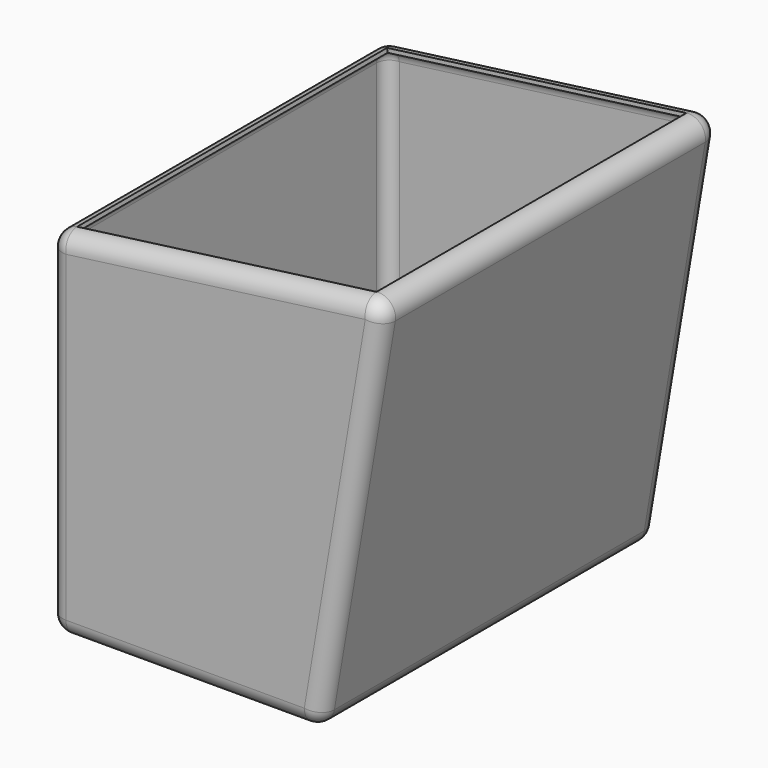
from build123d import *

# Parameters (mm, degrees)
F1_DEPTH = 125
F3_R     = 10
F4_T     = -2.5


# Not quite as in the source:
# - a shell that OpenCascade refuses in one call is made with other operations: the cavity is built on its own and cut out


with BuildPart() as f1:
    # F0 (on Front) → F1 (new body)
    with BuildSketch(Plane.XZ):
        Polygon((206.0437292722, 62.0864819473), (6.2040649354, 35.4162448123), (6.2040649354, -174.5837551877), (166.2040649354, -174.5837551877), align=None)
    extrude(amount=F1_DEPTH)

    # F2: F1 across plane


with BuildPart() as f1_1:
    add(f1.part)
    add(f1.part.mirror(Plane.XZ))

    # F3
    f3_edges = [f1_1.edges().sort_by_distance(p)[0] for p in [
        (106.123897, -125, 48.751363),
        (206.043729, 0, 62.086482),
        (186.123897, -125, -56.248637),
        (6.204065, -125, -69.583755),
        (86.204065, -125, -174.583755),
        (166.204065, 0, -174.583755),
        (106.123897, 125, 48.751363),
        (6.204065, 0, 35.416245),
        (186.123897, 125, -56.248637),
        (6.204065, 125, -69.583755),
        (86.204065, 125, -174.583755),
        (6.204065, 0, -174.583755),
    ]]
    fillet(f3_edges, radius=F3_R)

    # F4: a shell. OpenCascade refuses it in one call, so the cavity is built on its own and cut out:
    # the body offset inwards by the wall thickness, plus a prism from it out through each open face.
    f4_core = offset(f1_1.part, amount=F4_T, mode=Mode.PRIVATE)
    f4_exits = [f4_core.faces().sort_by_distance(p)[0] for p in [
        (104.076238, 0, 45.955921),
    ]]
    add(f4_core, mode=Mode.SUBTRACT)
    extrude(f4_exits, amount=-F4_T, mode=Mode.SUBTRACT)


solid = f1_1.part
